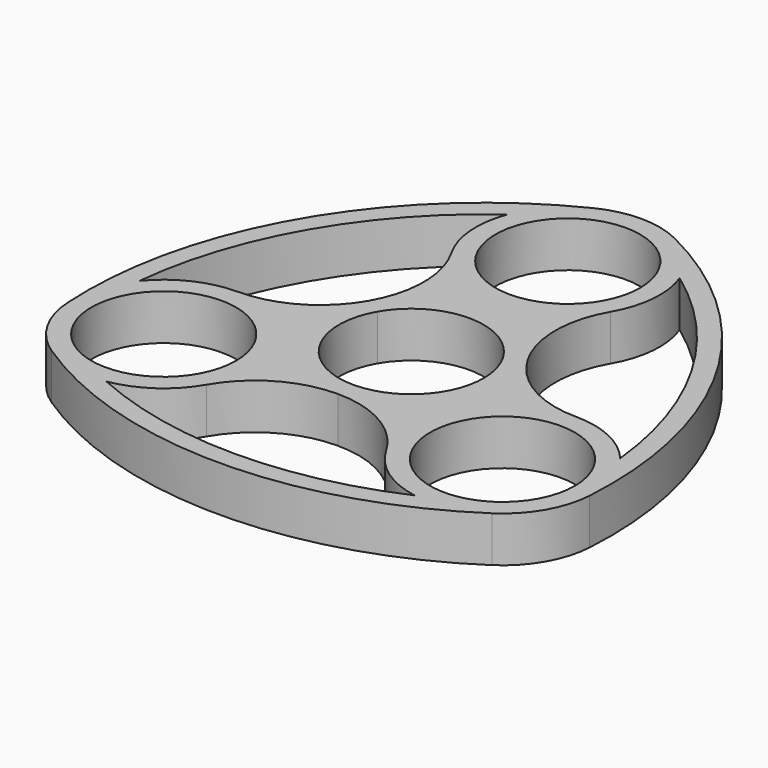
from build123d import *

# Parameters (mm, degrees)
F0_R            = 11.1
F1_DEPTH        = 7
F2_COUNT        = 3
F4_DEPTH        = 7
F4_COPIES_COUNT = 3


# Not quite as in the source:
# - a pattern or mirror of a feature is missing from the dataset's text; its kind, count and spacing are read off the source's solid


with BuildPart() as f1:
    # F0 (on Top) → F1 (new body)
    with BuildSketch(Plane.XY):
        with BuildLine():
            ThreePointArc((-9.612881982, 5.55), (0, 11.1), (9.612881982, 5.55))
            Line((9.612881982, 5.55), (12.2109581934, 7.05))
            ThreePointArc((12.2109581934, 7.05), (10.0807621135, 15), (12.2109581934, 22.95))
            ThreePointArc((12.2109581934, 22.95), (0, 44.1), (-12.2109581934, 22.95))
            ThreePointArc((-12.2109581934, 22.95), (-10.0807621135, 15), (-12.2109581934, 7.05))
            Line((-12.2109581934, 7.05), (-9.612881982, 5.55))
        make_face()
        with Locations((0, 30)):
            Circle(F0_R, mode=Mode.SUBTRACT)
    extrude(amount=F1_DEPTH)

    # F2: F1 ×3 about axis
    f2_axis = Axis((0, 0, 0), (0, 0, 1))


with BuildPart() as f1_1:
    add(f1.part)
    for i in range(1, F2_COUNT):
        add(f1.part.rotate(f2_axis, i * 360 / F2_COUNT))

    # F3 (on face) → F4 (join)
    with BuildSketch(Plane.XY):
        with BuildLine():
            Line((36.8595294383, -6.0299151903), (40.0530223584, -15.8840201358))
            ThreePointArc((40.0530223584, -15.8840201358), (31.9933329124, 18.4713593692), (6.2705462274, 42.6289449286))
            ThreePointArc((6.2705462274, 42.6289449286), (10.4711494103, 39.4427236552), (13.2077049817, 34.9362464602))
            ThreePointArc((13.2077049817, 34.9362464602), (29.395256701, 16.9713593692), (36.8595294383, -6.0299151903))
        make_face()
    f4 = extrude(amount=F4_DEPTH)

    # F4_copies: F4 ×3 about axis
    f4_copies_axis = Axis((0, 0, 0), (0, 0, 1))
    for i in range(1, F4_COPIES_COUNT):
        add(f4.rotate(f4_copies_axis, i * 360 / F4_COPIES_COUNT))


solid = f1_1.part
